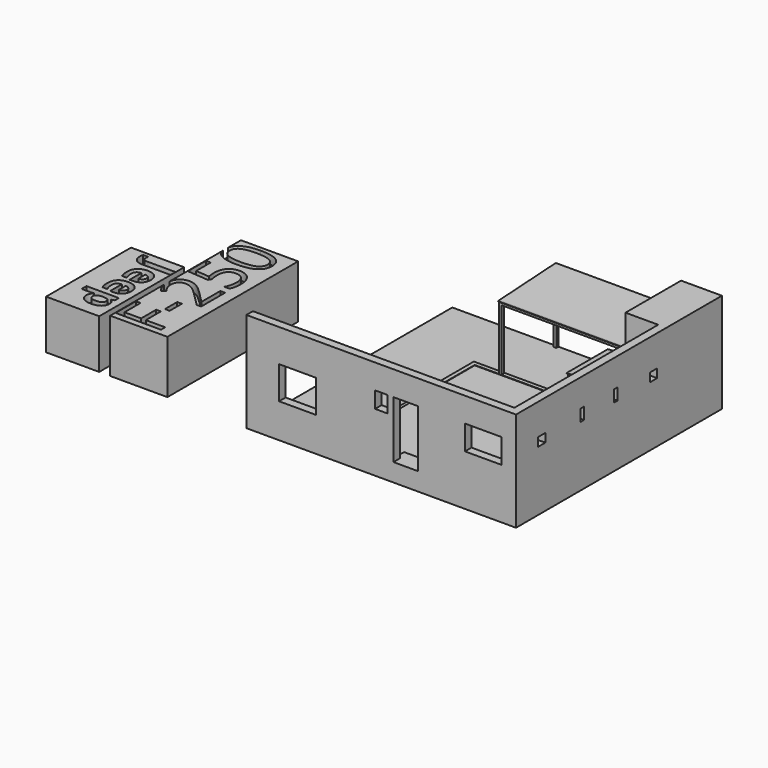
from build123d import *

# Parameters (mm, degrees)
F1_DEPTH       = 304.8
F2_W           = 5.08
F2_H           = 152.4
F3_DEPTH       = 127
F4_W           = 114.3
F4_H           = 101.6
F4_W_2         = 38.1
F4_H_2         = 50.8
F4_H_3         = 76.2
F4_W_3         = 76.2
F4_H_4         = 177.8
F5_DEPTH       = 25.4
F6_W           = 101.6
F6_H           = 50.8
F7_DEPTH       = 31.75
F8_W           = 25.4
F8_H           = 25.4
F9_DEPTH       = 101.6
F10_W          = 5.08
F10_H          = 127
F11_DEPTH      = 25.4
F12_W          = 838.2
F12_H          = 800.1
F13_DEPTH      = 5.08
F14_W          = 88.9
F14_H          = 25.4
F15_DEPTH      = 101.6
F17_DEPTH      = 12.7
F18_W          = 28.0128717422
F18_H          = 26.9354581833
F18_W_2        = 12.9290223122
F18_H_2        = 36.6322100163
F19_DEPTH      = 25.4
F20_W          = 165.1
F20_H          = 330.2
F21_DEPTH      = 152.4
F22_TEXT_SIZE  = 128.3812783658
F23_DEPTH      = 25.4
F24_W          = 177.8
F24_H          = 508
F25_DEPTH      = 165.1
F26_TEXT_SIZE  = 197.809686055
F27_DEPTH      = 25.4
F30_DEPTH      = 11.43
F31_W          = 12.7
F31_H          = 127
F32_DEPTH      = 12.7
F33_W          = 127.0357439709
F33_H          = 6.35
F34_DEPTH      = 15.24
F37_START      = 165.1
F36_W          = 152.4
F36_H          = 160.8582
F36_W_2        = 135.4836
F36_H_2        = 143.9418
F37_DEPTH      = 4.2418
F35_W          = 8.4582
F35_H          = 8.4582
F38_DEPTH      = 165.1
F40_DEPTH      = 160.8582
F41_W          = 44.45
F41_H          = 19.05
F42_DEPTH      = 152.4
F44_DEPTH      = 19.05
F47_START      = 203.2
F46_W          = 389.4582
F46_H          = 220.98
F46_W_2        = 372.5418
F46_H_2        = 204.0636
F47_DEPTH      = 4.2418
F45_W          = 8.4582
F45_H          = 8.4582
F48_DEPTH      = 203.2
F50_DEPTH      = 381
F50_DEPTH_BACK = 8.4582


# Not quite as in the source:
# - Text() gives the source's letters only with a copy of the font that has no kerning and outlines rounded to 1/6400 em; it was checked with that copy


with BuildPart() as f1:
    # F0 (on Top) → F1 (new body)
    with BuildSketch(Plane.XY):
        Polygon((0, 25.4), (0, 0), (146.7380461541, 0), (838.2, 0), (838.2, 25.4), (838.2, 192.8434281291), (838.2, 584.2), (838.2, 800.1), (711.2, 800.1), (711.2, 584.2), (812.8, 584.2), (812.8, 25.4), (25.4, 25.4), align=None)
    extrude(amount=F1_DEPTH)

    # F2 (on face) → F3 (join)
    with BuildSketch(Plane(origin=(711.2, 0, 0), x_dir=(0, -1, 0), z_dir=(-1, 0, 0))):
        with Locations((-797.56, 76.2)):
            Rectangle(F2_W, F2_H)
    extrude(amount=F3_DEPTH)

    # F4 (on face) → F5 (cut, through all)
    with BuildSketch(Plane(origin=(0, 25.4, 0), x_dir=(-1, 0, 0), z_dir=(0, 1, 0))):
        with Locations((-158.75, 152.4)):
            Rectangle(F4_W, F4_H)
        with Locations((-419.1, 203.2)):
            Rectangle(F4_W_2, F4_H_2)
        with Locations((-736.6, 190.5)):
            Rectangle(F4_W, F4_H_3)
        with Locations((-495.3, 139.7)):
            Rectangle(F4_W_3, F4_H_4)
    extrude(amount=-F5_DEPTH, mode=Mode.SUBTRACT)

    # F6 (on face) → F7 (join)
    with BuildSketch(Plane(origin=(0, 25.4, 0), x_dir=(-1, 0, 0), z_dir=(0, 1, 0))):
        with Locations((-495.3, 25.4)):
            Rectangle(F6_W, F6_H)
    extrude(amount=F7_DEPTH)

    # F8 (on face) → F9 (join, through all)
    with BuildSketch(Plane(origin=(444.5, 0, 0), x_dir=(0, -1, 0), z_dir=(-1, 0, 0))):
        with Locations((-69.85, 12.7)):
            Rectangle(F8_W, F8_H)
    extrude(amount=-F9_DEPTH)

    # F10 (on face) → F11 (join)
    with BuildSketch(Plane(origin=(0, 25.4, 0), x_dir=(-1, 0, 0), z_dir=(0, 1, 0))):
        with Locations((-2.54, 63.5)):
            Rectangle(F10_W, F10_H)
    extrude(amount=F11_DEPTH)

    # F12 (on face) → F13 (join)
    with BuildSketch(Plane(origin=(0, 0, 0), x_dir=(1, 0, 0), z_dir=(0, 0, -1))):
        with Locations((419.1, -400.05)):
            Rectangle(F12_W, F12_H)
    extrude(amount=F13_DEPTH)

    # F14 (on face) → F15 (join)
    with BuildSketch(Plane.XZ.offset(-584.2)):
        with Locations((768.35, 12.7)):
            Rectangle(F14_W, F14_H)
    extrude(amount=F15_DEPTH)

    # F16 (on face) → F17 (join)
    with BuildSketch(Plane.XY):
        Polygon((233.68, 591.82), (233.68, 25.4), (246.38, 25.4), (246.38, 579.12), (406.4, 579.12), (812.8, 579.12), (812.8, 591.82), (711.2, 591.82), align=None)
    extrude(amount=F17_DEPTH)

    # F18 (on face) → F19 (cut, through all)
    with BuildSketch(Plane(origin=(812.8, 0, 0), x_dir=(0, -1, 0), z_dir=(-1, 0, 0))):
        with Locations((-100.0905707479, 194.9580013752)):
            Rectangle(F18_W, F18_H)
        with Locations((-534.2900753021, 194.9580013752)):
            Rectangle(F18_W, F18_H)
        with Locations((-387.7612054348, 200.8838057518)):
            Rectangle(F18_W_2, F18_H_2)
        with Locations((-257.3936283588, 200.8838057518)):
            Rectangle(F18_W_2, F18_H_2)
    extrude(amount=-F19_DEPTH, mode=Mode.SUBTRACT)

    # F31 (on face) → F32 (cut)
    with BuildSketch(Plane.XY.offset(12.7)):
        with Locations((240.03, 302.26)):
            Rectangle(F31_W, F31_H)
    extrude(amount=-F32_DEPTH, mode=Mode.SUBTRACT)


with BuildPart() as f21:
    # F20 (on Top) → F21 (new body)
    with BuildSketch(Plane.XY):
        with Locations((-540.0967398967, 165.1)):
            Rectangle(F20_W, F20_H)
    extrude(amount=F21_DEPTH)

    # F22 (on face) → F23 (cut)
    with BuildSketch(Plane.XY.offset(152.4)):
        with Locations(Location((-549.98126032, 308.8669721949), (0, 0, -90))):
            Text('Jeep', F22_TEXT_SIZE, font='Open Sans', font_style=FontStyle.BOLD, text_align=(TextAlign.LEFT, TextAlign.BOTTOM))
    extrude(amount=-F23_DEPTH, mode=Mode.SUBTRACT)


with BuildPart() as f25:
    # F24 (on Top) → F25 (new body)
    with BuildSketch(Plane.XY):
        with Locations((-334.4333264497, 254)):
            Rectangle(F24_W, F24_H)
    extrude(amount=F25_DEPTH)

    # F26 (on face) → F27 (cut)
    with BuildSketch(Plane.XY.offset(165.1)):
        with Locations(Location((-280.9103524901, 0), (0, 0, 90))):
            Text('F-250', F26_TEXT_SIZE, font='Open Sans', text_align=(TextAlign.LEFT, TextAlign.BOTTOM))
    extrude(amount=-F27_DEPTH, mode=Mode.SUBTRACT)


with BuildPart() as f30:
    # F29 (on offset) → F30 (new body)
    with BuildSketch(Plane.XY):
        Polygon((723.9, 482.6), (723.9, 579.12), (246.38, 579.12), (246.38, 25.4), (444.5, 25.4), (444.5, 82.55), (546.1000000007, 82.55), (546.1, 25.4), (812.8, 25.4), (812.8, 482.6), align=None)
    extrude(amount=F30_DEPTH)


with BuildPart() as f34:
    # F33 (on face) → F34 (new body)
    with BuildSketch(Plane(origin=(246.38, 0, 0), x_dir=(0, -1, 0), z_dir=(-1, 0, 0))):
        with Locations((-302.26, 3.175)):
            Rectangle(F33_W, F33_H)
    extrude(amount=F34_DEPTH)


with BuildPart() as f37:
    # F36 (on face) → F37 (new body)
    with BuildSketch(Plane.XY.offset(11.43).offset(F37_START)):
        with Locations((736.6, 503.7709)):
            Rectangle(F36_W, F36_H)
        with Locations((736.6, 503.7709)):
            Rectangle(F36_W_2, F36_H_2, mode=Mode.SUBTRACT)
    extrude(amount=F37_DEPTH)

    # F35 (on face) → F38 (join, through all)
    with BuildSketch(Plane.XY.offset(11.43)):
        with Locations((664.6291, 579.9709)):
            Rectangle(F35_W, F35_H)
        with Locations((808.5709, 579.9709)):
            Rectangle(F35_W, F35_H)
        with Locations((664.6291, 427.5709)):
            Rectangle(F35_W, F35_H)
        with Locations((808.5709, 427.5709)):
            Rectangle(F35_W, F35_H)
    extrude(amount=F38_DEPTH)

    # F39 (on face) → F40 (join, through all)
    with BuildSketch(Plane.XZ.offset(-423.3418)):
        Polygon((660.4, 186.2082922458), (660.4, 180.7718), (664.6418, 180.7718), (664.6418, 186.5576212329), (734.7793347359, 192.3337242951), (734.7793347359, 180.7718), (738.4206652641, 180.7718), (738.4206652641, 192.6336022491), (808.5582, 198.4097053112), (808.5582, 180.7718), (812.8, 180.7718), (812.8, 199.8218), (660.4, 187.2710579475), (656.0712666431, 186.914569655), (656.1582, 185.8589632587), align=None)
    extrude(amount=-F40_DEPTH)


with BuildPart() as f42:
    # F41 (on face) → F42 (new body)
    with BuildSketch(Plane.XY.offset(11.43)):
        with Locations((741.2338345218, 392.9807841778)):
            Rectangle(F41_W, F41_H)
    extrude(amount=F42_DEPTH)

    # F43 (on face) → F44 (cut, through all)
    with BuildSketch(Plane.XZ.offset(-383.4557841778)):
        with BuildLine():
            ThreePointArc((741.2338345217, 163.83), (753.520430158, 154.3439644792), (747.4525245918, 140.0567035706))
            Line((747.4525245918, 140.0567035706), (747.4525245918, 138.43))
            Line((747.4525245918, 138.43), (763.4588345218, 138.43))
            Line((763.4588345218, 138.43), (763.4588345218, 163.83))
            Line((763.4588345218, 163.83), (741.2338345217, 163.83))
        make_face()
        with BuildLine():
            ThreePointArc((735.0151444519, 140.0567035706), (728.9472388856, 154.3439644791), (741.2338345217, 163.83))
            Line((741.2338345217, 163.83), (719.0088345218, 163.83))
            Line((719.0088345218, 163.83), (719.0088345218, 138.43))
            Line((719.0088345218, 138.43), (735.0151444519, 138.43))
            Line((735.0151444519, 138.43), (735.0151444519, 140.0567035706))
        make_face()
        Polygon((735.6635332108, 11.43), (719.0088345218, 138.43), (719.0088345218, 11.43), align=None)
        Polygon((763.4588345218, 11.43), (763.4588345218, 138.43), (746.8041358329, 11.43), align=None)
    extrude(amount=-F44_DEPTH, mode=Mode.SUBTRACT)


with BuildPart() as f47:
    # F46 (on face) → F47 (new body)
    with BuildSketch(Plane.XY.offset(F47_START)):
        with Locations((516.4709, 689.61)):
            Rectangle(F46_W, F46_H)
        with Locations((516.4709, 689.61)):
            Rectangle(F46_W_2, F46_H_2, mode=Mode.SUBTRACT)
    extrude(amount=F47_DEPTH)

    # F45 (on face) → F48 (join, through all)
    with BuildSketch(Plane.XY):
        with Locations((706.9709, 795.8709)):
            Rectangle(F45_W, F45_H)
        with Locations((706.9709, 583.3491)):
            Rectangle(F45_W, F45_H)
        with Locations((325.9709, 583.3491)):
            Rectangle(F45_W, F45_H)
        with Locations((325.9709, 795.8709)):
            Rectangle(F45_W, F45_H)
    extrude(amount=F48_DEPTH)

    # F49 (on face) → F50 (join, two sides)
    with BuildSketch(Plane.YZ.offset(330.2)) as f50_sk:
        Polygon((579.12, 212.7719564562), (579.12, 207.4418), (583.3618, 207.4418), (583.3618, 213.0149496537), (687.4891, 218.9799233854), (687.4891, 207.4418), (691.7309, 207.4418), (691.7309, 219.2229165829), (795.8582, 225.1878903145), (795.8582, 207.4418), (800.1, 207.4418), (800.1, 226.4918), (579.12, 213.8328729441), (574.8176237657, 213.586409613), (574.8782, 212.5289632587), align=None)
    extrude(amount=F50_DEPTH)
    extrude(f50_sk.sketch, amount=-F50_DEPTH_BACK)


solid = Compound([f1.part, f21.part, f25.part, f30.part, f34.part, f37.part, f42.part, f47.part])
